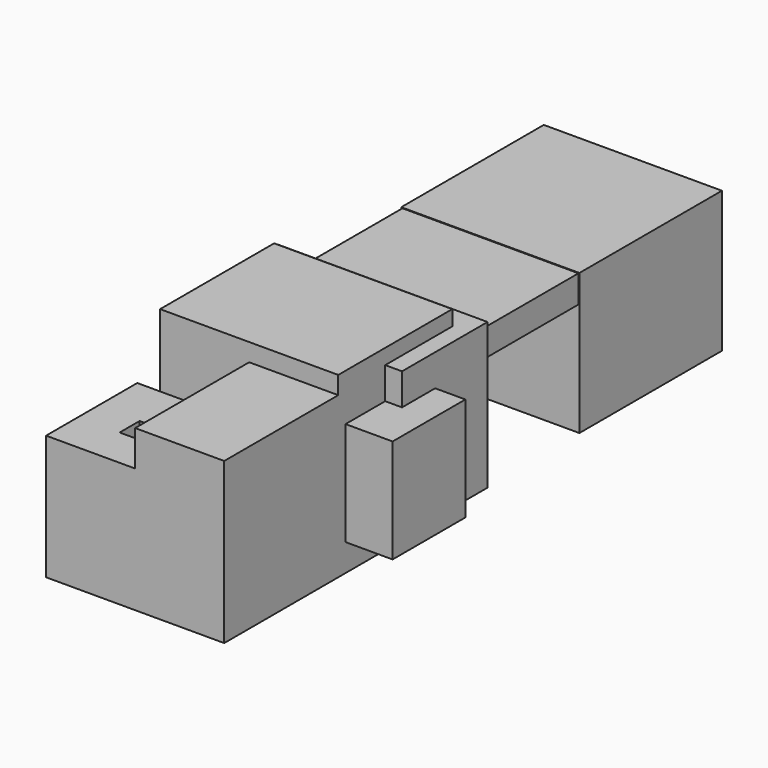
from build123d import *

# Parameters (mm, degrees)
F1_DEPTH  = 127
F2_DEPTH  = 114.3
F3_DEPTH  = 88.9
F6_DEPTH  = 76.2
F8_W      = 64.8522339761
F8_H      = 74.062012136
F9_DEPTH  = 38.1
F10_T     = -2.54
F11_W     = 125.4833117127
F11_H     = 19.5707902312
F12_DEPTH = 101.6
F14_W     = 127
F14_H     = 100.4699997724
F15_DEPTH = 127


# Not quite as in the source:
# - a shell that OpenCascade refuses in one call is made with other operations: the cavity is built on its own and cut out


with BuildPart() as f1:
    # F0 (on Top) → F1 (new body)
    with BuildSketch(Plane.XY):
        Polygon((27.6681821086, 78.8052295411), (-99.3318178914, 78.8052295411), (-99.3318178914, -22.7947704589), (-35.8318178914, -22.7947704589), (27.6681821086, -22.7947704589), align=None)
    extrude(amount=F1_DEPTH)

    # F0 (on Top) → F2 (join)
    with BuildSketch(Plane.XY):
        Polygon((27.6681821086, -124.3947704589), (27.6681821086, -22.7947704589), (-35.8318178914, -22.7947704589), (-35.8318178914, -95.8602428436), (-35.8318178914, -124.3947704589), align=None)
    extrude(amount=F2_DEPTH)

    # F0 (on Top) → F3 (join)
    with BuildSketch(Plane.XY):
        Polygon((-35.8318178914, -124.3947704589), (-35.8318178914, -95.8602428436), (-69.7213560343, -95.8602428436), (-69.7213560343, -85.9395861626), (-69.7213560343, -78.0614241958), (-50.7554039359, -78.0614241958), (-50.7554039359, -43.129093945), (-99.3318178914, -43.129093945), (-99.3318178914, -124.3947704589), align=None)
    extrude(amount=F3_DEPTH)

    # F5 (on offset) → F6 (join)
    with BuildSketch(Plane.XZ.offset(-95.25)):
        Polygon((-109.9954843521, 12.5446757302), (27.7675427496, 12.5446757302), (39.663515985, 12.1609345078), (39.663515985, 116.1547526717), (-109.9954843521, 116.1547526717), align=None)
    extrude(amount=F6_DEPTH)

    # F8 (on offset) → F9 (join)
    with BuildSketch(Plane.YZ.offset(61.214)):
        with Locations((16.1268953234, 56.4830191433)):
            Rectangle(F8_W, F8_H)
    extrude(amount=-F9_DEPTH)

    # F10: a shell. OpenCascade refuses it in one call, so the cavity is built on its own and cut out:
    # the body offset inwards by the wall thickness, plus a prism from it out through each open face.
    f10_core = offset(f1.part, amount=F10_T, kind=Kind.INTERSECTION, mode=Mode.PRIVATE)
    f10_exits = [f10_core.faces().sort_by_distance(p)[0] for p in [
        (-52.776587, -98.400243, 44.45),
    ]]
    add(f10_core, mode=Mode.SUBTRACT)
    extrude(f10_exits, amount=-F10_T, mode=Mode.SUBTRACT)

    # F11 (on offset) → F12 (join)
    with BuildSketch(Plane.XZ.offset(-95.25)):
        with Locations((-39.538461715, 90.2522318065)):
            Rectangle(F11_W, F11_H)
    extrude(amount=-F12_DEPTH)

    # F14 (on offset) → F15 (join)
    with BuildSketch(Plane.XZ.offset(-196.85)):
        with Locations((-39.6279752942, 50.2349998862)):
            Rectangle(F14_W, F14_H)
    extrude(amount=-F15_DEPTH)


solid = f1.part
